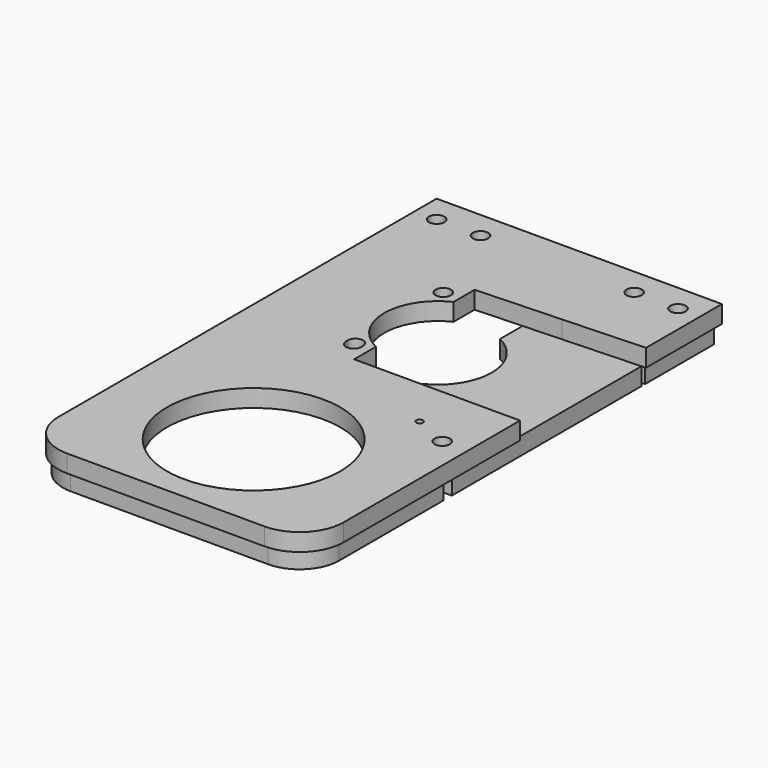
from build123d import *

# Parameters (mm, degrees)
F0_R     = 39.5
F0_R_2   = 3.5
F0_W     = 75.5830052443
F0_H     = 21
F1_DEPTH = 8
F2_R     = 20
F3_R     = 1.5
F3_W     = 40.198237868
F3_H     = 8.9987739231
F3_W_2   = 8.2853332109
F3_H_2   = 18.0666130036
F4_DEPTH = 8
F5_R     = 1.5
F6_DEPTH = 25
F5_R_2   = 3.5
F7_DEPTH = 8
F8_DEPTH = 25


# Not quite as in the source:
# - a feature names something its author has since deleted; it is built from what else it names


with BuildPart() as f1:
    # F0 (on Top) → F1 (new body)
    with BuildSketch(Plane.XY):
        with BuildLine():
            Line((44.5193349518, 39.5479659047), (-85.4806650482, 39.5479659047))
            Line((-85.4806650482, 39.5479659047), (-85.4806650482, -95.9520340953))
            Line((-85.4806650482, -95.9520340953), (-85.4806650482, -195.9520340953))
            Line((-85.4806650482, -195.9520340953), (44.5193349518, -195.9520340953))
            Line((44.5193349518, -195.9520340953), (44.5193349518, -96.4520340953))
            Line((44.5193349518, -96.4520340953), (-31.0636702925, -96.4520340953))
            Line((-31.0636702925, -96.4520340953), (-31.0636702925, -75.4520340953))
            Line((-31.0636702925, -75.4520340953), (-31.0636702925, -63.0484138893))
            ThreePointArc((-31.0636702925, -63.0484138893), (-44.9806650482, -40.9520340953), (-31.0636702925, -18.8556543013))
            Line((-31.0636702925, -18.8556543013), (-31.0636702925, -6.8642294387))
            Line((-31.0636702925, -6.8642294387), (-31.0636702925, 14.5479659047))
            Line((-31.0636702925, 14.5479659047), (6.7278323296, 14.5479659047))
            Line((6.7278323296, 14.5479659047), (44.5193349518, 14.5479659047))
            Line((44.5193349518, 14.5479659047), (44.5193349518, 39.5479659047))
        make_face()
        with Locations((-20.4806650482, -145.9520340953)):
            Circle(F0_R, mode=Mode.SUBTRACT)
        with Locations((32.9533093033, -105.3044921878)):
            Circle(F0_R_2, mode=Mode.SUBTRACT)
        with BuildLine():
            ThreePointArc((-34.9806650482, -66.4520340953), (-38.4806650482, -69.9520340953), (-41.9806650482, -66.4520340953))
            Line((-41.9806650482, -66.4520340953), (-41.9806650482, -65.4520340953))
            ThreePointArc((-41.9806650482, -65.4520340953), (-38.4806650482, -61.9520340953), (-34.9806650482, -65.4520340953))
            Line((-34.9806650482, -65.4520340953), (-34.9806650482, -66.4520340953))
        make_face(mode=Mode.SUBTRACT)
        with Locations((-75.4806650482, 27.0479659047)):
            Circle(F0_R_2, mode=Mode.SUBTRACT)
        with Locations((-55.4806650482, 27.0479659047)):
            Circle(F0_R_2, mode=Mode.SUBTRACT)
        with Locations((-38.4806650482, -15.4520340953)):
            Circle(F0_R_2, mode=Mode.SUBTRACT)
        with Locations((14.5193349518, 27.0479659047)):
            Circle(F0_R_2, mode=Mode.SUBTRACT)
        with Locations((34.5193349518, 27.0479659047)):
            Circle(F0_R_2, mode=Mode.SUBTRACT)
        with Locations((6.7278323296, -85.9520340953)):
            Rectangle(F0_W, F0_H)
        Polygon((44.5193349518, -3.7052528509), (44.5193349518, 14.5479659047), (6.7278323296, 14.5479659047), (7.5552909452, -5.2501576775), align=None)
        Polygon((7.5552909452, -5.2501576775), (6.7278323296, 14.5479659047), (-31.0636702925, 14.5479659047), (-31.0636702925, -6.8642294387), align=None)
    extrude(amount=F1_DEPTH)

    # F2
    f2_edges = [f1.edges().sort_by_distance(p)[0] for p in [
        (-85.480665, -195.952034, 4),
        (44.519335, -195.952034, 4),
    ]]
    fillet(f2_edges, radius=F2_R)

    # F5 (on face) → F6 (cut)
    with BuildSketch(Plane(origin=(0, 0, 0), x_dir=(1, 0, 0), z_dir=(0, 0, -1))):
        with Locations((17.0758515596, 98.3283445239)):
            Circle(F5_R)
    extrude(amount=-F6_DEPTH, mode=Mode.SUBTRACT)


with BuildPart() as f4:
    # F3 (on face) → F4 (new body)
    with BuildSketch(Plane(origin=(0, 0, 0), x_dir=(1, 0, 0), z_dir=(0, 0, -1))):
        Polygon((39.5193349518, -29.7293737531), (39.5193349518, -34.5479659047), (34.0944491327, -34.5479659047), (3.2112498302, -34.5479659047), (-36.9869880378, -34.5479659047), (-73.1572136283, -34.5479659047), (-80.4806650482, -34.5479659047), (-80.4806650482, -29.9261137843), (-80.4806650482, -3.7473780103), (-83.4806650482, -3.7473780103), (-83.4806650482, -37.5479659047), (42.5193349518, -37.5479659047), (42.5193349518, 1.7870964078), (39.5193349518, 1.7870964078), (39.5193349518, -1.7495956272), (39.5193349518, -19.8162086308), align=None)
        with BuildLine():
            Line((-83.4806650482, -3.7473780103), (-80.4806650482, -3.7473780103))
            Line((-80.4806650482, -3.7473780103), (-80.4806650482, 175.9520340953))
            ThreePointArc((-80.4806650482, 175.9520340953), (-76.087266766, 186.5586358131), (-65.4806650482, 190.9520340953))
            Line((-65.4806650482, 190.9520340953), (-61.6005832804, 190.9520340953))
            ThreePointArc((-61.6005832804, 190.9520340953), (-60.8013042068, 191.1827220917), (-60.0020251332, 190.9520340953))
            Line((-60.0020251332, 190.9520340953), (-20.4806650482, 190.9520340953))
            Line((-20.4806650482, 190.9520340953), (16.6160973065, 190.9520340953))
            ThreePointArc((16.6160973065, 190.9520340953), (17.4153763801, 191.1827220917), (18.2146554537, 190.9520340953))
            Line((18.2146554537, 190.9520340953), (24.5193349518, 190.9520340953))
            ThreePointArc((24.5193349518, 190.9520340953), (35.1259366696, 186.5586358131), (39.5193349518, 175.9520340953))
            Line((39.5193349518, 175.9520340953), (39.5193349518, 116.5885478258))
            Line((39.5193349518, 116.5885478258), (42.5193349518, 116.5885478258))
            Line((42.5193349518, 116.5885478258), (42.5193349518, 175.9520340953))
            ThreePointArc((42.5193349518, 175.9520340953), (37.2472570131, 188.6799561567), (24.5193349518, 193.9520340953))
            Line((24.5193349518, 193.9520340953), (-65.4806650482, 193.9520340953))
            ThreePointArc((-65.4806650482, 193.9520340953), (-78.2085871096, 188.6799561567), (-83.4806650482, 175.9520340953))
            Line((-83.4806650482, 175.9520340953), (-83.4806650482, -3.7473780103))
        make_face()
        with BuildLine():
            Line((24.5193349518, 190.9520340953), (32.0193349518, 183.4520340953))
            Line((32.0193349518, 183.4520340953), (39.5193349518, 175.9520340953))
            ThreePointArc((39.5193349518, 175.9520340953), (35.1259366696, 186.5586358131), (24.5193349518, 190.9520340953))
        make_face()
        with BuildLine():
            Line((16.6160973065, 190.9520340953), (-20.4806650482, 190.9520340953))
            Line((-20.4806650482, 190.9520340953), (32.0193349518, 183.4520340953))
            Line((32.0193349518, 183.4520340953), (24.5193349518, 190.9520340953))
            Line((24.5193349518, 190.9520340953), (18.2146554537, 190.9520340953))
            ThreePointArc((18.2146554537, 190.9520340953), (18.7285630786, 190.4076639478), (18.9153763801, 189.6827220917))
            ThreePointArc((18.9153763801, 189.6827220917), (16.6904345239, 188.3695353932), (16.6160973065, 190.9520340953))
        make_face()
        Polygon((39.5193349518, 175.9520340953), (32.0193349518, 183.4520340953), (32.0193349518, 116.5885478258), (39.5193349518, 116.5885478258), align=None)
        with Locations((35.5012193322, 130.6999841353)):
            Circle(F3_R, mode=Mode.SUBTRACT)
        with Locations((35.5012193322, 168.9480393119)):
            Circle(F3_R, mode=Mode.SUBTRACT)
        with BuildLine():
            ThreePointArc((-65.4806650482, 190.9520340953), (-76.087266766, 186.5586358131), (-80.4806650482, 175.9520340953))
            Line((-80.4806650482, 175.9520340953), (-72.9806650482, 183.4520340953))
            Line((-72.9806650482, 183.4520340953), (-65.4806650482, 190.9520340953))
        make_face()
        Polygon((-80.4806650482, 175.9520340953), (-80.4806650482, -3.7473780103), (-72.9806650482, -3.7473780103), (-72.9806650482, 183.4520340953), align=None)
        with Locations((-76.232790947, 23.5664832836)):
            Circle(F3_R, mode=Mode.SUBTRACT)
        with Locations((-76.232790947, 97.0494272842)):
            Circle(F3_R, mode=Mode.SUBTRACT)
        with Locations((-76.232790947, 156.2834084034)):
            Circle(F3_R, mode=Mode.SUBTRACT)
        with Locations((-16.8878691038, -30.0485789431)):
            Rectangle(F3_W, F3_H)
        with Locations((-28.3880401403, -29.805501923)):
            Circle(F3_R, mode=Mode.SUBTRACT)
        with Locations((-4.4237997708, -29.805501923)):
            Circle(F3_R, mode=Mode.SUBTRACT)
        with BuildLine():
            Line((-61.6005832804, 190.9520340953), (-65.4806650482, 190.9520340953))
            Line((-65.4806650482, 190.9520340953), (-72.9806650482, 183.4520340953))
            Line((-72.9806650482, 183.4520340953), (-20.4806650482, 190.9520340953))
            Line((-20.4806650482, 190.9520340953), (-60.0020251332, 190.9520340953))
            ThreePointArc((-60.0020251332, 190.9520340953), (-59.4881175083, 190.4076639478), (-59.3013042068, 189.6827220917))
            ThreePointArc((-59.3013042068, 189.6827220917), (-61.5262460629, 188.3695353932), (-61.6005832804, 190.9520340953))
        make_face()
        with Locations((35.3766683463, -10.782902129)):
            Rectangle(F3_W_2, F3_H_2)
        with Locations((35.5012193322, -10.2002834901)):
            Circle(F3_R, mode=Mode.SUBTRACT)
    extrude(amount=F4_DEPTH)


with BuildPart() as f7:
    # F5 (on face) → F7 (new body)
    with BuildSketch(Plane(origin=(0, 0, 0), x_dir=(1, 0, 0), z_dir=(0, 0, -1))):
        Polygon((42.5193349518, 3.788842451), (42.5193349518, 111.8137985468), (17.5193349518, 111.8137985468), (0, 75.4520340953), (-9.8976650482, 75.4520340953), (-9.8976650482, 5.9796004827), (0, 5.5659295515), align=None)
        with Locations((17.0758515596, 98.3283445239)):
            Circle(F5_R, mode=Mode.SUBTRACT)
        with Locations((32.9533093033, 105.3044921878)):
            Circle(F5_R_2, mode=Mode.SUBTRACT)
    extrude(amount=F7_DEPTH)

    # F0 (on Top) → F8 (cut)
    with BuildSketch(Plane.XY):
        with BuildLine():
            ThreePointArc((4.0193349518, -40.9520340953), (-7.4237440575, -20.2212161124), (-31.0636702925, -18.8556543013))
            Line((-31.0636702925, -18.8556543013), (-31.0636702925, -63.0484138893))
            ThreePointArc((-31.0636702925, -63.0484138893), (-7.4237440575, -61.6828520783), (4.0193349518, -40.9520340953))
        make_face()
    extrude(amount=-F8_DEPTH, mode=Mode.SUBTRACT)


solid = Compound([f1.part, f4.part, f7.part])
